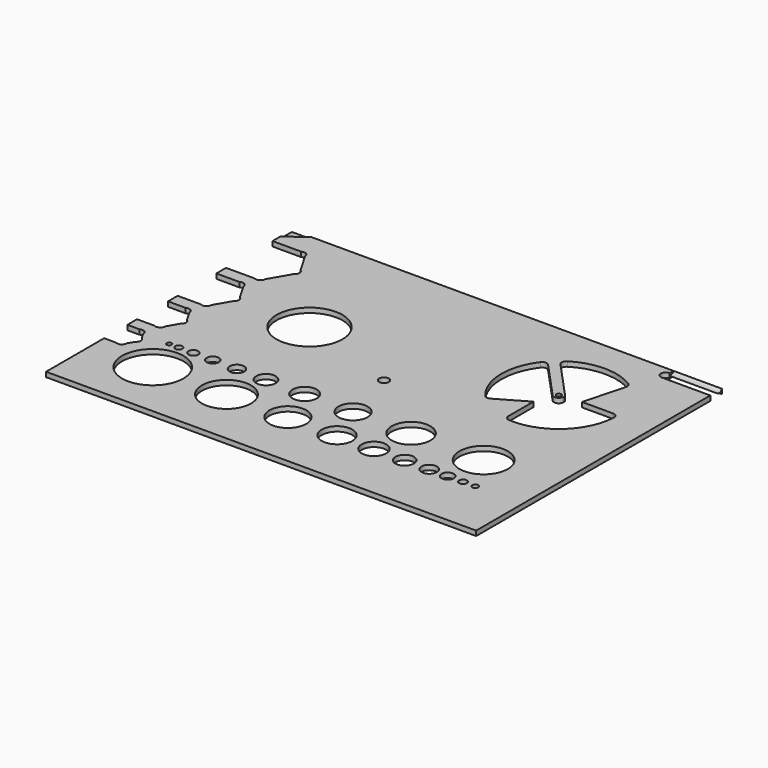
from build123d import *

# Parameters (mm, degrees)
F0_W          = 88.9
F0_H          = 63.5
F1_DEPTH      = 1
F5_DEPTH      = 25
F7_DEPTH      = 10
F8_R          = 5
F8_R_2        = 6.35
F8_R_3        = 5.08
F8_R_4        = 3.81
F8_R_5        = 3.175
F8_R_6        = 2.54
F8_R_7        = 1.905
F8_R_8        = 1.5875
F8_R_9        = 1.27
F8_R_10       = 0.79375
F8_R_11       = 0.635
F8_R_12       = 4
F8_R_13       = 3
F8_R_14       = 2.5
F8_R_15       = 2
F8_R_16       = 1.5
F8_R_17       = 1.25
F8_R_18       = 1
F8_R_19       = 0.75
F8_R_20       = 0.5
F8_R_21       = 6.82
F9_DEPTH      = 25
F11_DEPTH     = 0.375
F13_DEPTH     = 0.375
F14_T4_DEPTH  = 8.903123749
F14_T10_DEPTH = 8.903123749


# Not quite as in the source:
# - a fillet or chamfer that OpenCascade refuses, or shapes differently, is made with other operations: its cross-section is extruded or revolved along the edge and cut away or added
# - ends of sketch curves that miss each other by under 0.0002 mm in the source are joined


with BuildPart() as f1:
    # F0 (on Top) → F1 (new body)
    with BuildSketch(Plane.XY):
        with Locations((44.45, 31.75)):
            Rectangle(F0_W, F0_H)
    extrude(amount=F1_DEPTH)

    # F4 (on face) → F5 (cut)
    with BuildSketch(Plane.XY.offset(1)):
        with BuildLine():
            Line((78.9, 60.5), (88.9, 60.5))
            Line((88.9, 60.5), (88.9, 62.5))
            Line((88.9, 62.5), (78.9, 62.5))
            ThreePointArc((78.9, 62.5), (79.6071067812, 62.2071067812), (79.9, 61.5))
            ThreePointArc((79.9, 61.5), (79.6071067812, 60.7928932188), (78.9, 60.5))
        make_face()
        with BuildLine():
            ThreePointArc((78.9, 62.5), (77.9, 61.5), (78.9, 60.5))
            Line((78.9, 60.5), (78.9, 62.5))
        make_face()
        with BuildLine():
            Line((78.9, 62.5), (78.9, 60.5))
            ThreePointArc((78.9, 60.5), (79.6071067812, 60.7928932188), (79.9, 61.5))
            ThreePointArc((79.9, 61.5), (79.6071067812, 62.2071067812), (78.9, 62.5))
        make_face()
    extrude(amount=-F5_DEPTH, mode=Mode.SUBTRACT)

    # F6 (on face) → F7 (cut)
    with BuildSketch(Plane.YZ.offset(88.9)):
        with BuildLine():
            add(Edge.make_bspline(
                [(63.5, 0), (63.5, 0.5), (62.5, 0.5)],
                knots=[0, 0, 0, 1.5707963268, 1.5707963268, 1.5707963268], degree=2, weights=[1, 0.7071067812, 1]))
            Line((62.5, 0.5), (62.5, 0))
            Line((62.5, 0), (63.5, 0))
        make_face()
        with BuildLine():
            Line((63.5, 1), (62.5, 1))
            Line((62.5, 1), (62.5, 0.5))
            add(Edge.make_bspline(
                [(62.5, 0.5), (63.5, 0.5), (63.5, 1)],
                knots=[4.7123889804, 4.7123889804, 4.7123889804, 6.2831853072, 6.2831853072, 6.2831853072], degree=2, weights=[1, 0.7071067812, 1]))
        make_face()
    extrude(amount=-F7_DEPTH, mode=Mode.SUBTRACT)

    # F8 (on face) → F9 (cut)
    with BuildSketch(Plane.XY.offset(1)):
        with Locations((74.45, 20)):
            Circle(F8_R)
        with Locations((12.45, 12)):
            Circle(F8_R_2)
        with Locations((27.69, 12)):
            Circle(F8_R_3)
        with Locations((40.39, 12)):
            Circle(F8_R_4)
        with Locations((50.55, 12)):
            Circle(F8_R_5)
        with Locations((58.17, 12)):
            Circle(F8_R_6)
        with Locations((64.52, 12)):
            Circle(F8_R_7)
        with Locations((69.6, 12)):
            Circle(F8_R_8)
        with Locations((73.41, 12)):
            Circle(F8_R_9)
        with Locations((76.585, 12)):
            Circle(F8_R_10)
        with Locations((79.125, 12)):
            Circle(F8_R_11)
        with Locations((59.45, 20)):
            Circle(F8_R_12)
        with Locations((47.45, 20)):
            Circle(F8_R_13)
        with Locations((37.45, 20)):
            Circle(F8_R_14)
        with Locations((29.45, 20)):
            Circle(F8_R_15)
        with Locations((23.45, 20)):
            Circle(F8_R_16)
        with Locations((18.45, 20)):
            Circle(F8_R_17)
        with Locations((14.45, 20)):
            Circle(F8_R_18)
        with Locations((11.45, 20)):
            Circle(F8_R_19)
        with Locations((9.45, 20)):
            Circle(F8_R_20)
        with BuildLine():
            Line((0, 14.9999996647), (2.4641016151, 14.9999996647))
            ThreePointArc((2.4641016151, 14.9999996647), (3.4641016151, 14.9999996647), (3.9641016151, 15.8660250685))
            Line((3.9641016151, 15.8660250685), (4.6961524227, 17.1339742609))
            ThreePointArc((4.6961524227, 17.1339742609), (5.1961524227, 17.9999996647), (4.6961524227, 18.8660250685))
            Line((4.6961524227, 18.8660250685), (3.9641016151, 20.1339742609))
            ThreePointArc((3.9641016151, 20.1339742609), (3.4641016151, 20.9999996647), (2.4641016151, 20.9999996647))
            Line((2.4641016151, 20.9999996647), (0, 20.9999996647))
            Line((0, 20.9999996647), (-1.7320508076, 17.9999996647))
            Line((-1.7320508076, 17.9999996647), (0, 14.9999996647))
        make_face()
        with BuildLine():
            Line((-2.8867513459, 39.0000018477), (0, 34.0000018477))
            Line((0, 34.0000018477), (4.7735026919, 34.0000018477))
            ThreePointArc((4.7735026919, 34.0000018477), (5.2735026919, 33.8660272515), (5.7735026919, 34.0000018477))
            ThreePointArc((5.7735026919, 34.0000018477), (6.1395280957, 34.3660272515), (6.2735026919, 34.8660272515))
            Line((6.2735026919, 34.8660272515), (8.1602540378, 38.133976444))
            ThreePointArc((8.1602540378, 38.133976444), (8.6602540378, 39.0000018477), (8.1602540378, 39.8660272515))
            Line((8.1602540378, 39.8660272515), (6.2735026919, 43.133976444))
            ThreePointArc((6.2735026919, 43.133976444), (5.7735026919, 44.0000018477), (4.7735026919, 44.0000018477))
            Line((4.7735026919, 44.0000018477), (0, 44.0000018477))
            Line((0, 44.0000018477), (-2.8867513459, 39.0000018477))
        make_face()
        with BuildLine():
            Line((0, 23.4999991953), (3.6188021535, 23.4999991953))
            ThreePointArc((3.6188021535, 23.4999991953), (4.6188021535, 23.4999991953), (5.1188021535, 24.3660245991))
            Line((5.1188021535, 24.3660245991), (6.4282032303, 26.6339737916))
            ThreePointArc((6.4282032303, 26.6339737916), (6.9282032303, 27.4999991953), (6.4282032303, 28.3660245991))
            Line((6.4282032303, 28.3660245991), (5.1188021535, 30.6339737916))
            ThreePointArc((5.1188021535, 30.6339737916), (4.6188021535, 31.4999991953), (3.6188021535, 31.4999991953))
            Line((3.6188021535, 31.4999991953), (0, 31.4999991953))
            Line((0, 31.4999991953), (-2.3094010768, 27.4999991953))
            Line((-2.3094010768, 27.4999991953), (0, 23.4999991953))
        make_face()
        with BuildLine():
            Line((0, 46.5000011027), (5.9282032303, 46.5000011027))
            ThreePointArc((5.9282032303, 46.5000011027), (6.9282032303, 46.5000011027), (7.4282032303, 47.3660265065))
            Line((7.4282032303, 47.3660265065), (9.8923048454, 51.6339756989))
            ThreePointArc((9.8923048454, 51.6339756989), (10.3923048454, 52.5000011027), (9.8923048454, 53.3660265065))
            Line((9.8923048454, 53.3660265065), (7.4282032303, 57.6339756989))
            ThreePointArc((7.4282032303, 57.6339756989), (6.9282032303, 58.5000011027), (5.9282032303, 58.5000011027))
            Line((5.9282032303, 58.5000011027), (0, 58.5000011027))
            Line((0, 58.5000011027), (-3.4641016151, 52.5000011027))
            Line((-3.4641016151, 52.5000011027), (0, 46.5000011027))
        make_face()
        with BuildLine():
            ThreePointArc((75.9965413819, 55.4239037183), (69.7064402802, 57.2188103383), (63.4195722631, 55.4126120713))
            ThreePointArc((63.4195722631, 55.4126120713), (62.9586056452, 54.6985726023), (63.2134724878, 53.8877794854))
            Line((63.2134724878, 53.8877794854), (70.453229681, 46.0140204974))
            ThreePointArc((70.453229681, 46.0140204974), (70.6488055759, 45.7004057151), (70.7171076571, 45.3371716473))
            ThreePointArc((70.7171076571, 45.3371716473), (70.080341725, 44.4054737284), (68.9809856332, 44.6603227971))
            Line((68.9809856332, 44.6603227971), (61.74122844, 52.5340817851))
            ThreePointArc((61.74122844, 52.5340817851), (60.9546293112, 52.8559581533), (60.2044919449, 52.4564127647))
            ThreePointArc((60.2044919449, 52.4564127647), (57.8402849867, 44.9987414015), (60.6253238546, 37.6877978778))
            ThreePointArc((60.6253238546, 37.6877978778), (61.2175210997, 37.3466734256), (61.8905196516, 37.4655700956))
            Line((61.8905196516, 37.4655700956), (67.9713955599, 40.9763654382))
            Line((67.9713955599, 40.9763654382), (67.9713955599, 34.4811098251))
            ThreePointArc((67.9713955599, 34.4811098251), (68.2404614442, 33.7986617916), (68.9028661968, 33.4834607253))
            ThreePointArc((68.9028661968, 33.4834607253), (77.6018812733, 36.4487636459), (81.5833352867, 44.7321149393))
            ThreePointArc((81.5833352867, 44.7321149393), (81.3112334204, 45.4700985969), (80.5896132811, 45.7830261909))
            Line((80.5896132811, 45.7830261909), (74.1475280684, 45.7830385939))
            Line((74.1475280684, 45.7830385939), (76.4339684801, 54.3161503788))
            ThreePointArc((76.4339684801, 54.3161503788), (76.3981531684, 54.9422494851), (75.9965413819, 55.4239037183))
        make_face()
        with Locations((69.7171076571, 45.3371716473)):
            Circle(F8_R_20)
        with Locations((23.45, 38.750000298)):
            Circle(F8_R_21)
        with Locations((44.45, 31.75)):
            Circle(F8_R_18)
    extrude(amount=-F9_DEPTH, mode=Mode.SUBTRACT)

    # F10 (on face) → F11 (cut)
    with BuildSketch(Plane.XY.offset(1)):
        Polygon((0, 63.5), (0, 60.5), (4, 63.5), align=None)
    extrude(amount=-F11_DEPTH, mode=Mode.SUBTRACT)

    # F12 (on face) → F13 (cut)
    with BuildSketch(Plane(origin=(0, 0, 0), x_dir=(1, 0, 0), z_dir=(0, 0, -1))):
        Polygon((4, -63.5), (0, -60.5), (0, -63.5), align=None)
    extrude(amount=-F13_DEPTH, mode=Mode.SUBTRACT)

    # F14: fillet of radius 1 on 2 edges, made by hand


with BuildPart() as f14_tool2:
    # F14_s3 → F14_t4 (new body)
    with BuildSketch(Plane(origin=(27.4787505004, 20.6090628753, 0), x_dir=(0, 0, 1), z_dir=(0.8, 0.6, 0))):
        with BuildLine():
            ThreePointArc((1, -48.4), (0.7236121811, -48.7476120479), (0.625, -49.1806247498))
            Line((0.625, -49.1806247498), (0.625, -48.4))
            Line((0.625, -48.4), (1, -48.4))
        make_face()
    extrude(amount=F14_T4_DEPTH)

    split(bisect_by=Plane.YZ, keep=Keep.TOP)

    split(bisect_by=Plane.XZ.offset(-63.5), keep=Keep.TOP)


with BuildPart() as f1_1:
    add(f1.part)

    # F14_t1: union F14_tool2
    add(f14_tool2.part)


with BuildPart() as f14_tool8:
    # F14_s9 → F14_t10 (new body)
    with BuildSketch(Plane(origin=(34.6012494996, 25.9509371247, 0), x_dir=(0, 0, 1), z_dir=(-0.8, -0.6, 0))):
        with BuildLine():
            ThreePointArc((0.375, 49.1806247498), (0.2763878189, 48.7476120479), (0, 48.4))
            Line((0, 48.4), (0.375, 48.4))
            Line((0.375, 48.4), (0.375, 49.1806247498))
        make_face()
    extrude(amount=F14_T10_DEPTH)

    split(bisect_by=Plane.YZ, keep=Keep.TOP)

    split(bisect_by=Plane.XZ.offset(-63.5), keep=Keep.TOP)


with BuildPart() as f1_2:
    add(f1_1.part)

    # F14_t7: union F14_tool8
    add(f14_tool8.part)


solid = f1_2.part
